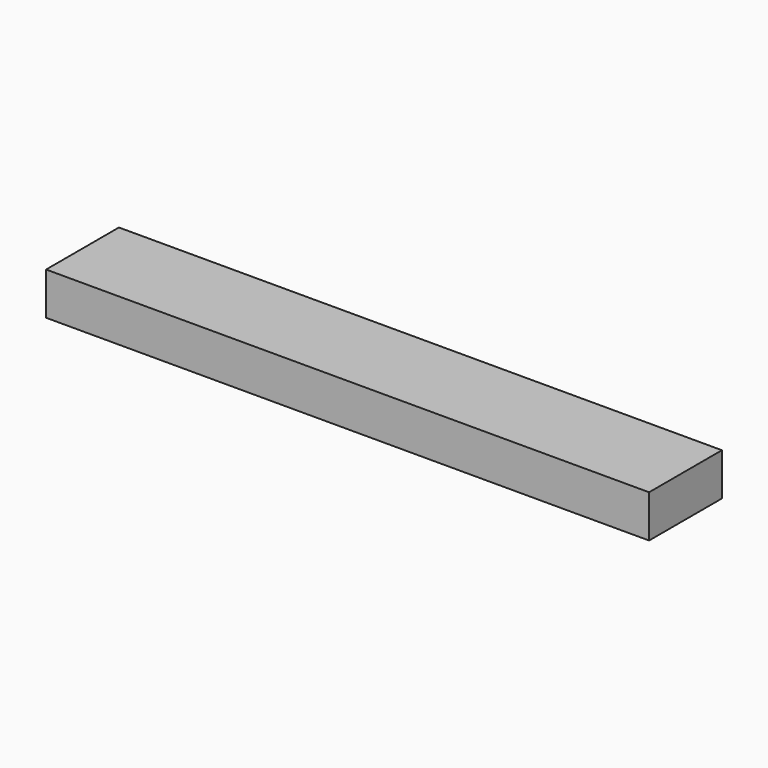
from build123d import *

# Parameters (mm, degrees)
F1_E0_W  = 29.8
F1_E0_H  = 4.5
F2_DEPTH = 2.1


with BuildPart() as f2:
    # F1_E0 (on explicit) → F2 (new body)
    with BuildSketch(Plane(origin=(-44.1323819277, 0, 0), x_dir=(1, 0, 0), z_dir=(0, 0, 1))):
        with Locations((14.9, 2.25)):
            Rectangle(F1_E0_W, F1_E0_H)
    extrude(amount=-F2_DEPTH)


solid = f2.part
